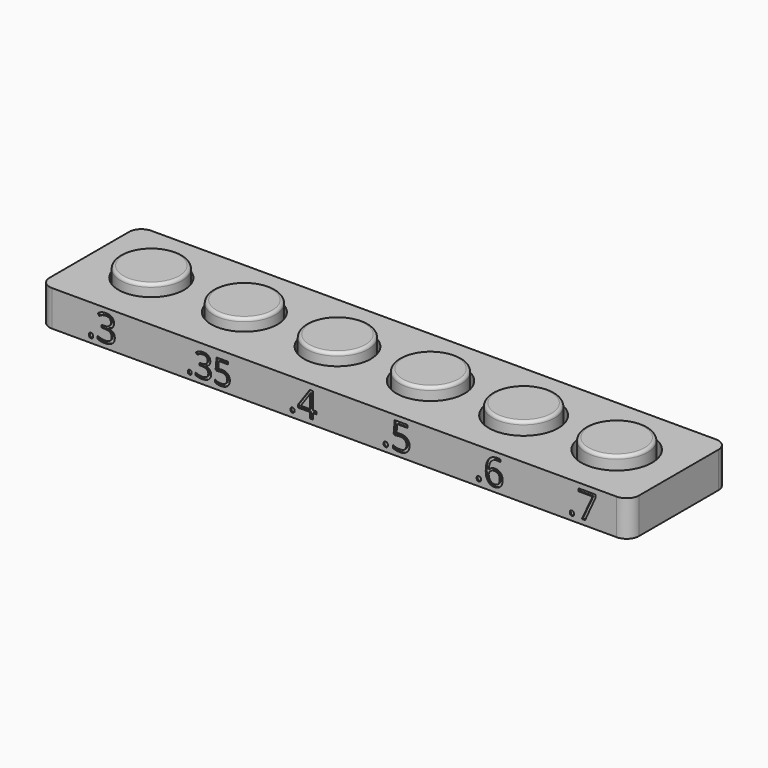
from build123d import *

# Parameters (mm, degrees)
F0_W           = 95
F0_H           = 20
F0_R           = 5.3
F0_R_2         = 5.35
F0_R_3         = 5.4
F0_R_4         = 5.5
F0_R_5         = 5.6
F0_R_6         = 5.7
F1_DEPTH       = 5.76003
F0_R_7         = 5
F2_DEPTH       = 7.5
F3_TEXT_SIZE   = 5.9237319511
F3_TEXT_SIZE_2 = 5.2933392148
F3_TEXT_SIZE_3 = 5.6647194194
F3_TEXT_SIZE_4 = 5.9160658162
F3_TEXT_SIZE_5 = 5.8554437328
F3_TEXT_SIZE_6 = 5.8694057227
F4_DEPTH       = 0.2
F5_R           = 0.5
F5_2_R         = 0.5
F5_3_R         = 0.5
F5_4_R         = 0.5
F5_5_R         = 0.5
F5_6_R         = 0.5
F6_R           = 2


# Not quite as in the source:
# - Text() gives the source's letters only with a copy of the font that has no kerning and outlines rounded to 1/6400 em; it was checked with that copy


with BuildPart() as f1:
    # F0 (on Top) → F1 (new body)
    with BuildSketch(Plane.XY):
        Rectangle(F0_W, F0_H)
        with Locations((-37.5, 0)):
            Circle(F0_R, mode=Mode.SUBTRACT)
        with Locations((-22.5, 0)):
            Circle(F0_R_2, mode=Mode.SUBTRACT)
        with Locations((-7.5, 0)):
            Circle(F0_R_3, mode=Mode.SUBTRACT)
        with Locations((7.5, 0)):
            Circle(F0_R_4, mode=Mode.SUBTRACT)
        with Locations((22.5, 0)):
            Circle(F0_R_5, mode=Mode.SUBTRACT)
        with Locations((37.5, 0)):
            Circle(F0_R_6, mode=Mode.SUBTRACT)
    extrude(amount=F1_DEPTH)

    # F3 (on face) → F4 (cut)
    with BuildSketch(Plane.XZ.offset(10)):
        with Locations((-40, 0.76003)):
            Text('.3', F3_TEXT_SIZE, font='Open Sans', text_align=(TextAlign.LEFT, TextAlign.BOTTOM))
        with Locations((-24, 0.76003)):
            Text('.35', F3_TEXT_SIZE_2, font='Open Sans', text_align=(TextAlign.LEFT, TextAlign.BOTTOM))
        with Locations((-7.5, 0.76003)):
            Text('.4', F3_TEXT_SIZE_3, font='Open Sans', text_align=(TextAlign.LEFT, TextAlign.BOTTOM))
        with Locations((7.5, 0.76003)):
            Text('.5', F3_TEXT_SIZE_4, font='Open Sans', text_align=(TextAlign.LEFT, TextAlign.BOTTOM))
        with Locations((22.5, 0.76003)):
            Text('.6', F3_TEXT_SIZE_5, font='Open Sans', text_align=(TextAlign.LEFT, TextAlign.BOTTOM))
        with Locations((37.5, 0.76003)):
            Text('.7', F3_TEXT_SIZE_6, font='Open Sans', text_align=(TextAlign.LEFT, TextAlign.BOTTOM))
    extrude(amount=-F4_DEPTH, mode=Mode.SUBTRACT)

    # F6
    f6_edges = [f1.edges().sort_by_distance(p)[0] for p in [
        (47.5, 10, 2.880015),
        (47.5, -10, 2.880015),
        (-47.5, -10, 2.880015),
        (-47.5, 10, 2.880015),
    ]]
    fillet(f6_edges, radius=F6_R)


with BuildPart() as f2:
    # F0 (on Top) → F2 (new body)
    with BuildSketch(Plane.XY):
        with Locations((-37.5, 0)):
            Circle(F0_R_7)
    extrude(amount=F2_DEPTH)

    # F5
    f5_edges = [f2.edges().sort_by_distance(p)[0] for p in [
        (-42.5, 0, 7.5),
        (-42.5, 0, 0),
    ]]
    fillet(f5_edges, radius=F5_R)


with BuildPart() as f2b:
    # F0 (on Top) → F2, piece 2 (new body)
    with BuildSketch(Plane.XY):
        with Locations((-22.5, 0)):
            Circle(F0_R_7)
    extrude(amount=F2_DEPTH)

    # F5#2
    f5_2_edges = [f2b.edges().sort_by_distance(p)[0] for p in [
        (-27.5, 0, 7.5),
        (-27.5, 0, 0),
    ]]
    fillet(f5_2_edges, radius=F5_2_R)


with BuildPart() as f2c:
    # F0 (on Top) → F2, piece 3 (new body)
    with BuildSketch(Plane.XY):
        with Locations((-7.5, 0)):
            Circle(F0_R_7)
    extrude(amount=F2_DEPTH)

    # F5#3
    f5_3_edges = [f2c.edges().sort_by_distance(p)[0] for p in [
        (-12.5, 0, 7.5),
        (-12.5, 0, 0),
    ]]
    fillet(f5_3_edges, radius=F5_3_R)


with BuildPart() as f2d:
    # F0 (on Top) → F2, piece 4 (new body)
    with BuildSketch(Plane.XY):
        with Locations((7.5, 0)):
            Circle(F0_R_7)
    extrude(amount=F2_DEPTH)

    # F5#4
    f5_4_edges = [f2d.edges().sort_by_distance(p)[0] for p in [
        (2.5, 0, 7.5),
        (2.5, 0, 0),
    ]]
    fillet(f5_4_edges, radius=F5_4_R)


with BuildPart() as f2e:
    # F0 (on Top) → F2, piece 5 (new body)
    with BuildSketch(Plane.XY):
        with Locations((22.5, 0)):
            Circle(F0_R_7)
    extrude(amount=F2_DEPTH)

    # F5#5
    f5_5_edges = [f2e.edges().sort_by_distance(p)[0] for p in [
        (17.5, 0, 7.5),
        (17.5, 0, 0),
    ]]
    fillet(f5_5_edges, radius=F5_5_R)


with BuildPart() as f2f:
    # F0 (on Top) → F2, piece 6 (new body)
    with BuildSketch(Plane.XY):
        with Locations((37.5, 0)):
            Circle(F0_R_7)
    extrude(amount=F2_DEPTH)

    # F5#6
    f5_6_edges = [f2f.edges().sort_by_distance(p)[0] for p in [
        (32.5, 0, 7.5),
        (32.5, 0, 0),
    ]]
    fillet(f5_6_edges, radius=F5_6_R)


solid = Compound([f1.part, f2.part, f2b.part, f2c.part, f2d.part, f2e.part, f2f.part])
